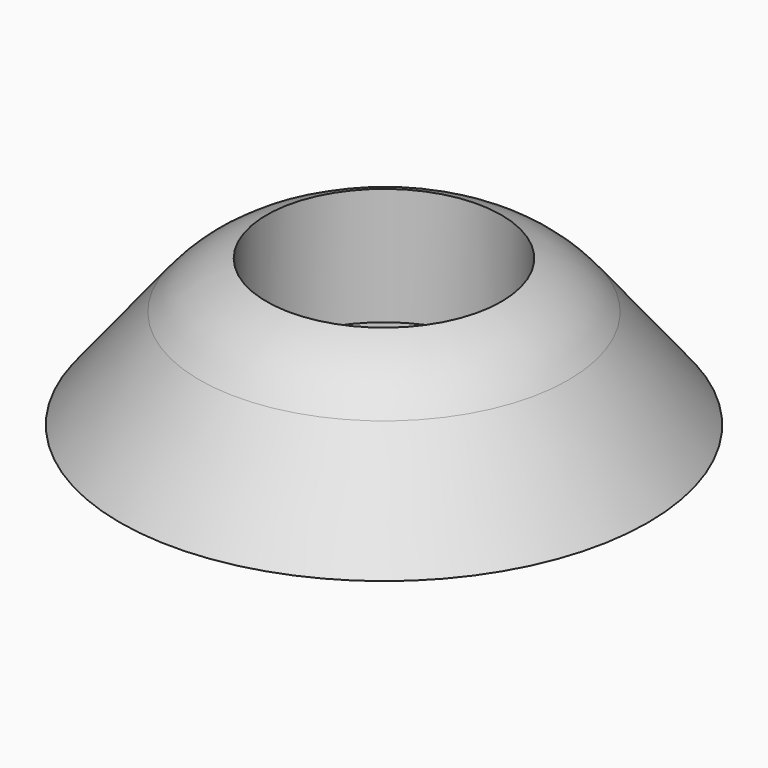
from build123d import *

# Parameters (mm, degrees)
F2_R     = 1.75
F3_DEPTH = 1.001


# Not quite as in the source:
# - a fillet or chamfer that OpenCascade refuses, or shapes differently, is made with other operations: its cross-section is extruded or revolved along the edge and cut away or added


with BuildPart() as f1:
    # F0 (on Front) → F1 (revolve)
    with BuildSketch(Plane.XZ):
        Polygon((0, 1), (0, 0), (9, 0), (5, 5), (4, 5), (4, 1), align=None)
    revolve(axis=Axis((0, 0, 2.5), (0, 0, 1)))

    # F2 (on face) → F3 (cut, through all)
    with BuildSketch(Plane.XY.offset(1)):
        Circle(F2_R)
    extrude(amount=-F3_DEPTH, mode=Mode.SUBTRACT)

    # F4: fillet of radius 5 on 1 edges, made by hand

    # F4_s1 → F4_t2 (revolve, cut)
    with BuildSketch(Plane.XZ):
        with BuildLine():
            ThreePointArc((6.2858644818, 3.3926693977), (5.2575025417, 4.3592707998), (4, 5))
            Line((4, 5), (5, 5))
            Line((5, 5), (6.2858644818, 3.3926693977))
        make_face()
    revolve(axis=Axis((0, 0, 5), (0, 0, 1)), mode=Mode.SUBTRACT)


solid = f1.part
